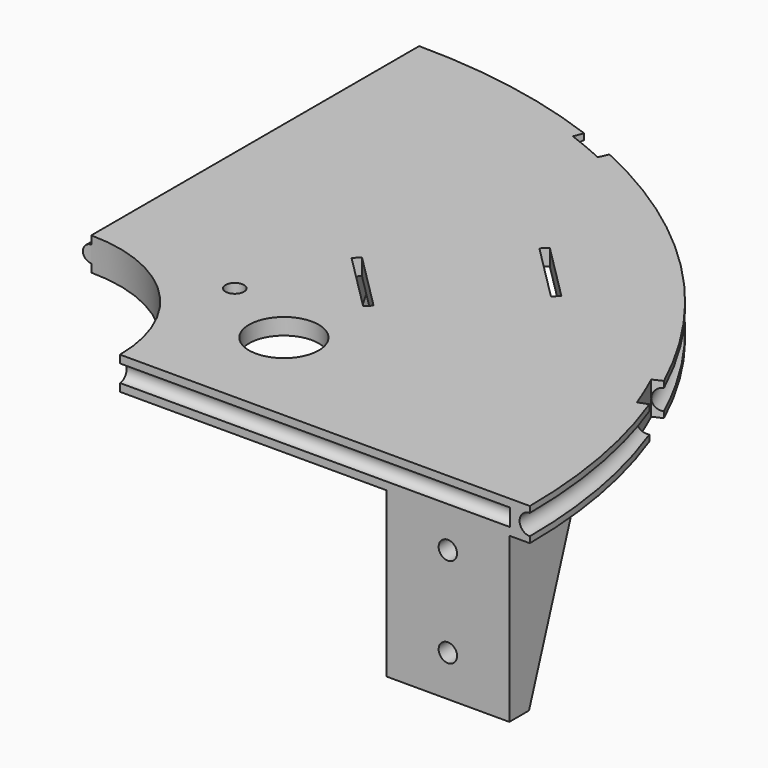
from build123d import *

# Parameters (mm, degrees)
F0_R         = 2.25
F1_DEPTH     = 8
F4_R         = 2.5
F6_W         = 30
F6_H         = 20
F6_W_2       = 20
F6_H_2       = 30
F7_DEPTH     = 40
F8_W         = 15
F8_H         = 14
F8_W_2       = 14
F8_H_2       = 15
F9_DEPTH     = 40
F10_SIZE2    = 39.99999
F10_SIZE     = 13.99999
F10_2_SIZE2  = 39.99999
F10_2_SIZE   = 13.99999
F11_R        = 2.25
F12_DEPTH    = 25
F14_R        = 2.25
F15_DEPTH    = 25
F17_DEPTH    = 25
F19_DEPTH    = 8.0010001
F22_R        = 2
F25_DEPTH    = 48.001
F26_R        = 2.1
F28_R        = 8.5
F29_DEPTH    = 8.0010001
F31_DEPTH    = 4
F32_T1_DEPTH = 4


# Not quite as in the source:
# - a fillet or chamfer that OpenCascade refuses, or shapes differently, is made with other operations: its cross-section is extruded or revolved along the edge and cut away or added
# - two fillets or chamfers of one size are made in one step
# - a fillet or chamfer is up to 0.001 mm smaller than in the source, because OpenCascade refuses the exact size


with BuildPart() as f1:
    # F0 (on Top) → F1 (new body)
    with BuildSketch(Plane.XY):
        with BuildLine():
            Line((35, 0), (135, 0))
            ThreePointArc((135, 0), (95.4594154602, 95.4594154602), (0, 135))
            Line((0, 135), (0, 35))
            ThreePointArc((0, 35), (24.7487373415, 24.7487373415), (35, 0))
        make_face()
        with Locations((35, 35)):
            Circle(F0_R, mode=Mode.SUBTRACT)
    extrude(amount=F1_DEPTH)

    # F5: sweep along a path in F3
    with BuildLine(Plane.XY.offset(4)) as f5_path:
        CenterArc((0, 0), 135, 0, 360)
    # F4 (on face) → F5 (sweep, cut)
    with BuildSketch(Plane.XZ):
        with Locations((135, 4)):
            Circle(F4_R)
    sweep(path=f5_path.line, mode=Mode.SUBTRACT)

    # F6 (on face) → F7 (join)
    with BuildSketch(Plane(origin=(0, 0, 0), x_dir=(1, 0, 0), z_dir=(0, 0, -1))):
        with Locations((115, -10)):
            Rectangle(F6_W, F6_H)
        with Locations((10, -115)):
            Rectangle(F6_W_2, F6_H_2)
    extrude(amount=F7_DEPTH)

    # F8 (on face) → F9 (cut)
    with BuildSketch(Plane(origin=(0, 0, -40), x_dir=(1, 0, 0), z_dir=(0, 0, -1))):
        with Locations((115, -13)):
            Rectangle(F8_W, F8_H)
        with Locations((13, -115)):
            Rectangle(F8_W_2, F8_H_2)
    extrude(amount=-F9_DEPTH, mode=Mode.SUBTRACT)

    # F10 (size 14 and 40 in the source; OpenCascade refuses exactly that, so slightly less here)
    f10_edges = [f1.edges().sort_by_distance(p)[0] for p in [
        (103.75, 20, -40),
        (126.25, 20, -40),
    ]]
    f10_side = f1.faces().sort_by_distance((129.639445, 10, -40))[0]
    chamfer(f10_edges, length=F10_SIZE, length2=F10_SIZE2, reference=f10_side)

    # F10#2 (size 14 and 40 in the source; OpenCascade refuses exactly that, so slightly less here)
    f10_2_edges = [f1.edges().sort_by_distance(p)[0] for p in [
        (20, 103.75, -40),
        (20, 126.25, -40),
    ]]
    f10_2_side = f1.faces().sort_by_distance((19.639445, 103.75, -40))[0]
    chamfer(f10_2_edges, length=F10_2_SIZE, length2=F10_2_SIZE2, reference=f10_2_side)

    # F11 (on face) → F12 (cut)
    with BuildSketch(Plane(origin=(0, 6, 0), x_dir=(-1, 0, 0), z_dir=(0, 1, 0))):
        with Locations((-115, -8)):
            Circle(F11_R)
        with Locations((-115, -30)):
            Circle(F11_R)
    extrude(amount=-F12_DEPTH, mode=Mode.SUBTRACT)

    # F14 (on face) → F15 (cut)
    with BuildSketch(Plane.YZ.offset(6)):
        with Locations((115, -30)):
            Circle(F14_R)
        with Locations((115, -8)):
            Circle(F14_R)
    extrude(amount=-F15_DEPTH, mode=Mode.SUBTRACT)

    # F16 (on face) → F17 (cut)
    with BuildSketch(Plane.XY.offset(8)):
        with BuildLine():
            ThreePointArc((120.4496071259, 55.2099822787), (122.4117800348, 50.7110057948), (124.2059779255, 46.1424430169))
            Line((124.2059779255, 46.1424430169), (126.549486943, 47.0130551493))
            ThreePointArc((126.549486943, 47.0130551493), (124.7214362618, 51.6678172249), (122.7222412226, 56.2516800575))
            Line((122.7222412226, 56.2516800575), (120.4496071259, 55.2099822787))
        make_face()
        with BuildLine():
            Line((47.0017845491, 126.5536733928), (46.1313811315, 124.2100868484))
            ThreePointArc((46.1313811315, 124.2100868484), (50.7001036814, 122.416295838), (55.1992548973, 120.4545236128))
            Line((55.1992548973, 120.4545236128), (56.2407502727, 122.7272504734))
            ThreePointArc((56.2407502727, 122.7272504734), (51.6567094112, 124.7260372689), (47.0017845491, 126.5536733928))
        make_face()
    extrude(amount=-F17_DEPTH, mode=Mode.SUBTRACT)

    # F18 (on face) → F19 (cut, through all)
    with BuildSketch(Plane(origin=(0, 0, 0), x_dir=(1, 0, 0), z_dir=(0, 0, -1))):
        Polygon((44.5477272148, -58.6898628385), (45.9619407771, -60.1040764009), (60.1040764009, -45.9619407771), (58.6898628385, -44.5477272148), align=None)
        Polygon((84.1457069612, -70.0035713375), (70.0035713375, -84.1457069612), (71.4177848998, -85.5599205236), (85.5599205236, -71.4177848998), align=None)
    extrude(amount=-F19_DEPTH, mode=Mode.SUBTRACT)

    # F23: sweep along a path in F21
    with BuildLine(Plane(origin=(0, 0, 0), x_dir=(0, -1, 0), z_dir=(-1, 0, 0))) as f23_path:
        Line((-130, 4), (0, 4))
    # F22 (on Front) → F23 (sweep)
    with BuildSketch(Plane.XZ):
        with Locations((0, 4)):
            Circle(F22_R)
    sweep(path=f23_path.line)

    # F24 (on face) → F25 (cut, through all)
    with BuildSketch(Plane.XY.offset(8)):
        with BuildLine():
            ThreePointArc((0, 35), (-24.7487373415, -24.7487373415), (35, 0))
            ThreePointArc((35, 0), (24.7487373415, 24.7487373415), (0, 35))
        make_face()
    extrude(amount=-F25_DEPTH, mode=Mode.SUBTRACT)

    # F27: sweep along a path in F20
    with BuildLine(Plane.XZ) as f27_path:
        Line((0, 4), (130.2, 4))
    # F26 (on Right) → F27 (sweep, cut)
    with BuildSketch(Plane.YZ):
        with Locations((0, 4)):
            Circle(F26_R)
    sweep(path=f27_path.line, mode=Mode.SUBTRACT)

    # F28 (on face) → F29 (cut, through all)
    with BuildSketch(Plane(origin=(0, 0, 0), x_dir=(1, 0, 0), z_dir=(0, 0, -1))):
        with Locations((55, -25)):
            Circle(F28_R)
    extrude(amount=-F29_DEPTH, mode=Mode.SUBTRACT)

    # F30 (on face) → F31 (cut)
    with BuildSketch(Plane(origin=(0, 0, 0), x_dir=(1, 0, 0), z_dir=(0, 0, -1))):
        with BuildLine():
            Line((37, -40), (13, -40))
            ThreePointArc((13, -40), (9.4644660941, -41.4644660941), (8, -45))
            Line((8, -45), (8, -100))
            Line((8, -100), (20, -100))
            Line((20, -100), (20, -122.5))
            ThreePointArc((20, -122.5), (87.7674484077, -87.7674484077), (122.5, -20))
            Line((122.5, -20), (100, -20))
            Line((100, -20), (100, -8))
            Line((100, -8), (45, -8))
            ThreePointArc((45, -8), (41.4644660941, -9.4644660941), (40, -13))
            Line((40, -13), (40, -37))
            ThreePointArc((40, -37), (39.1213203436, -39.1213203436), (37, -40))
        make_face()
    extrude(amount=-F31_DEPTH, mode=Mode.SUBTRACT)

    # F32: fillet of radius 5 on 4 edges, made by hand

    # F32_s2 → F32_t1 (join)
    with BuildSketch(Plane.XY):
        with BuildLine():
            ThreePointArc((100, 13), (98.5355339059, 9.4644660941), (95, 8))
            Line((95, 8), (100, 8))
            Line((100, 8), (100, 13))
        make_face()
        with BuildLine():
            ThreePointArc((13, 100), (9.4644660941, 98.5355339059), (8, 95))
            Line((8, 95), (8, 100))
            Line((8, 100), (13, 100))
        make_face()
        with BuildLine():
            ThreePointArc((26.0493451107, 121.3576599119), (21.8572882373, 120.3578891664), (20, 116.469012365))
            Line((20, 116.469012365), (20, 122.5))
            ThreePointArc((20, 122.5), (23.0317559361, 121.9663405145), (26.0493451107, 121.3576599119))
        make_face()
        with BuildLine():
            ThreePointArc((121.3576599119, 26.0493451107), (120.3578891664, 21.8572882373), (116.469012365, 20))
            Line((116.469012365, 20), (122.5, 20))
            ThreePointArc((122.5, 20), (121.9663405145, 23.0317559361), (121.3576599119, 26.0493451107))
        make_face()
    extrude(amount=F32_T1_DEPTH)


solid = f1.part
